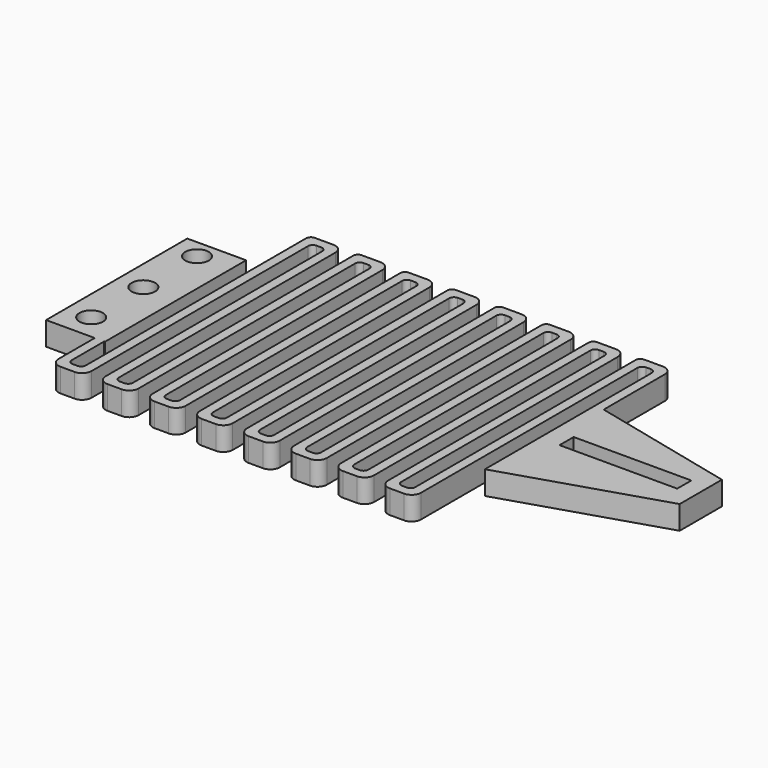
from build123d import *

# Parameters (mm, degrees)
F0_W      = 1.2
F0_H      = 0.8
F1_DEPTH  = 2
F2_R      = 0.4
F3_R      = 0.8
F11_DEPTH = 2
F14_DEPTH = 2
F15_R     = 1
F16_DEPTH = 2.001
F17_W     = 10
F17_H     = 1.5
F18_DEPTH = 2.001


with BuildPart() as f1:
    # F0 (on Top) → F1 (new body)
    with BuildSketch(Plane.XY):
        Polygon((8.5839435473, 25.4264183629), (8.5839435473, 13.2264183629), (9.3839435473, 13.2264183629), (9.3839435473, 26.2264183629), (6.5839435473, 26.2264183629), (6.5839435473, 2.0264183629), (6.5839435473, 1.2264183629), (7.3839435473, 1.2264183629), (7.3839435473, 25.4264183629), align=None)
        Polygon((4.5839435473, 1.2264183629), (5.3839435473, 1.2264183629), (5.3839435473, 2.0264183629), (5.3839435473, 14.2264183629), (4.5839435473, 14.2264183629), align=None)
        with Locations((5.9839435473, 1.6264183629)):
            Rectangle(F0_W, F0_H)
    extrude(amount=F1_DEPTH)

    # F2
    f2_edges = [f1.edges().sort_by_distance(p)[0] for p in [
        (7.383944, 25.426418, 1),
        (8.583944, 25.426418, 1),
        (5.383944, 2.026418, 1),
        (6.583944, 2.026418, 1),
        (6.583944, 26.226418, 1),
    ]]
    fillet(f2_edges, radius=F2_R)

    # F3
    f3_edges = [f1.edges().sort_by_distance(p)[0] for p in [
        (9.383944, 26.226418, 1),
        (7.383944, 1.226418, 1),
        (4.583944, 1.226418, 1),
    ]]
    fillet(f3_edges, radius=F3_R)


with BuildPart() as f4_1:
    # F4: copy of F1
    add(f1.part.moved(Location((4, 0, 0))))


with BuildPart() as f1_1:
    add(f1.part)

    # F5: union F4_1
    add(f4_1.part)


with BuildPart() as f6_1:
    # F6: copy of F1
    add(f1_1.part.moved(Location((8, 0, 0))))


with BuildPart() as f1_2:
    add(f1_1.part)

    # F7: union F6_1
    add(f6_1.part)


with BuildPart() as f8_1:
    # F8: copy of F1
    add(f1_2.part.moved(Location((16, 0, 0))))


with BuildPart() as f1_3:
    add(f1_2.part)

    # F9: union F8_1
    add(f8_1.part)

    # F10 (on face) → F11 (join)
    with BuildSketch(Plane.XY.offset(2)):
        Polygon((5.4478760238, 5.8683240786), (5.4478760238, 20.8683240786), (0.4478760238, 20.8683240786), (0.4478760238, 5.8683240786), (4.5839435473, 5.8683240786), (4.5839435473, 14.2264183629), (5.3839435473, 14.2264183629), (5.3839435473, 5.8683240786), align=None)
    extrude(amount=-F11_DEPTH)

    # F12: union 

    # F13 (on face) → F14 (join)
    with BuildSketch(Plane.XY.offset(2)):
        Polygon((49.8028248549, 15.969062224), (37.3839435473, 18.9353367689), (37.3839435473, 13.2264183629), (36.5839435473, 13.2264183629), (36.5839435473, 7.3133227415), (49.8028248549, 11.4841348702), align=None)
    extrude(amount=-F14_DEPTH)

    # F15 (on face) → F16 (cut, through all)
    with BuildSketch(Plane.XY.offset(2)):
        with Locations((2.5405562483, 19.2878898233)):
            Circle(F15_R)
        with Locations((2.5405562483, 13.5867726058)):
            Circle(F15_R)
        with Locations((2.5405562483, 8.0455001444)):
            Circle(F15_R)
    extrude(amount=-F16_DEPTH, mode=Mode.SUBTRACT)

    # F17 (on face) → F18 (cut, through all)
    with BuildSketch(Plane.XY.offset(2)):
        with Locations((43.2889471948, 13.8618260324)):
            Rectangle(F17_W, F17_H)
    extrude(amount=-F18_DEPTH, mode=Mode.SUBTRACT)


solid = f1_3.part
